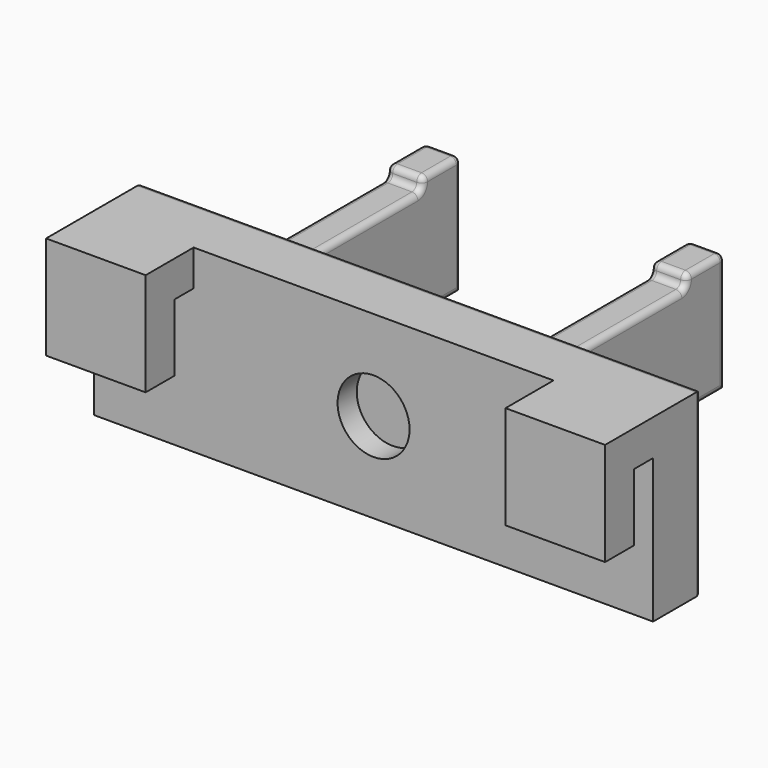
from build123d import *

# Parameters (mm, degrees)
F1_DEPTH = 23.3
F2_W     = 30
F2_H     = 8.6
F3_DEPTH = 5
F4_R     = 3
F5_DEPTH = 2
F7_DEPTH = 10
F8_W     = 12
F8_H     = 1
F9_DEPTH = 35.801
F10_R    = 0.49999


# Not quite as in the source:
# - a fillet or chamfer is up to 0.001 mm smaller than in the source, because OpenCascade refuses the exact size


with BuildPart() as f1:
    # F0 (on Right) → F1 (new body, symmetric)
    with BuildSketch(Plane.YZ):
        Polygon((-5, 12), (-5, 0), (0, 0), (0, 15), (-10, 15), (-10, 6.4), (-7, 6.4), (-7, 12), align=None)
    extrude(amount=F1_DEPTH, both=True)

    # F2 (on face) → F3 (cut, through all)
    with BuildSketch(Plane.XZ.offset(10)):
        with Locations((0, 10.7)):
            Rectangle(F2_W, F2_H)
    extrude(amount=-F3_DEPTH, mode=Mode.SUBTRACT)

    # F4 (on face) → F5 (cut)
    with BuildSketch(Plane.XZ.offset(5)):
        with Locations((0, 7.5)):
            Circle(F4_R)
    extrude(amount=-F5_DEPTH, mode=Mode.SUBTRACT)

    # F6 (on face) → F7 (join)
    with BuildSketch(Plane.XY.offset(15)):
        Polygon((-12.5, 16), (-12.5, 0), (-9.5, 0), (-9.5, 13), (-9.5, 16), align=None)
        Polygon((9.5, 13), (9.5, 0), (12.5, 0), (12.5, 16), (9.5, 16), align=None)
    extrude(amount=-F7_DEPTH)

    # F8 (on face) → F9 (cut, through all)
    with BuildSketch(Plane.YZ.offset(12.5)):
        with Locations((6, 14.5)):
            Rectangle(F8_W, F8_H)
    extrude(amount=-F9_DEPTH, mode=Mode.SUBTRACT)

    # F10 (radius 0.5 in the source; OpenCascade refuses exactly that, so slightly less here)
    f10_edges = [f1.edges().sort_by_distance(p)[0] for p in [
        (-9.5, 6, 14),
        (-9.5, 12, 14.5),
        (-9.5, 14, 15),
        (-9.5, 16, 10),
        (-9.5, 8, 5),
        (-9.5, 0, 9.5),
        (12.5, 6, 14),
        (12.5, 12, 14.5),
        (12.5, 14, 15),
        (12.5, 16, 10),
        (12.5, 8, 5),
        (12.5, 0, 9.5),
        (9.5, 14, 15),
        (9.5, 12, 14.5),
        (9.5, 6, 14),
        (9.5, 0, 9.5),
        (9.5, 8, 5),
        (9.5, 16, 10),
        (-12.5, 14, 15),
        (-12.5, 12, 14.5),
        (-12.5, 6, 14),
        (-12.5, 0, 9.5),
        (-12.5, 8, 5),
        (-12.5, 16, 10),
        (11, 12, 14),
        (-11, 12, 14),
        (-11, 16, 15),
        (-11, 12, 15),
        (11, 16, 15),
        (11, 12, 15),
        (0, 0, 0),
        (-23.3, 0, 7.5),
        (0, 0, 15),
        (23.3, 0, 7.5),
        (11, 0, 14),
        (11, 0, 5),
        (-11, 0, 14),
        (-11, 0, 5),
    ]]
    fillet(f10_edges, radius=F10_R)


solid = f1.part
